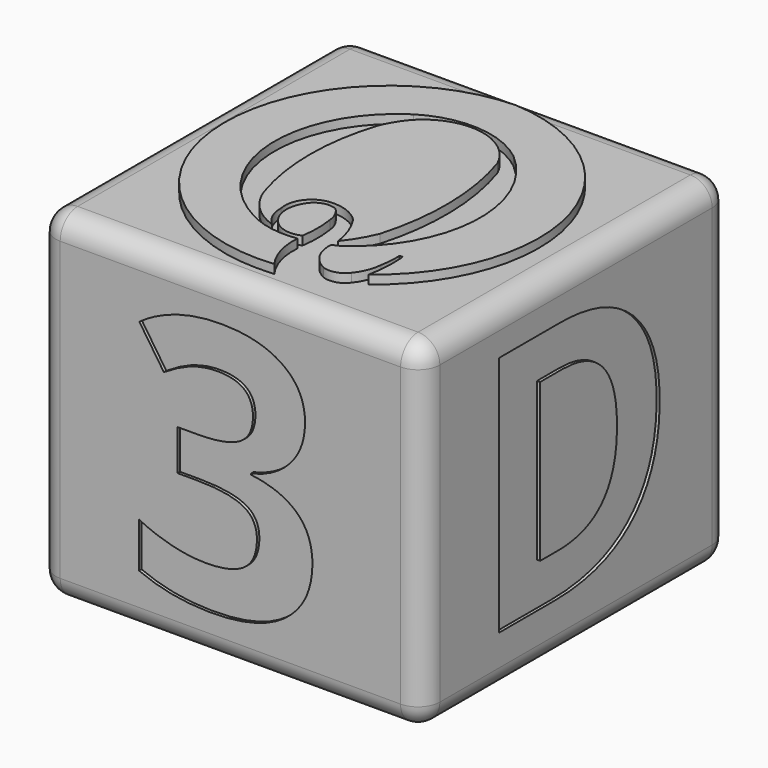
from build123d import *

# Parameters (mm, degrees)
F1_DEPTH      = 25
F4_DEPTH      = 55
F4_DEPTH_BACK = 23
F5_TEXT_SIZE  = 77.6406609496
F6_DEPTH      = 0.7
F7_TEXT_SIZE  = 80.3978016226
F8_DEPTH      = 0.7
F9_R          = 5


# Not quite as in the source:
# - Text() gives the source's letters only with a copy of the font that has no kerning and outlines rounded to 1/6400 em; it was checked with that copy


with BuildPart() as f1:
    # F0 (on Top) → F1 (new body)
    with BuildSketch(Plane.XY):
        with BuildLine():
            ThreePointArc((20.5675270408, -24.0095891058), (33.9110650067, 17.0205442488), (0, 43.6956547201))
            ThreePointArc((0, 43.6956547201), (-36.3351686492, 3.6568551313), (4.842115661, -31.3828539161))
            ThreePointArc((4.842115661, -31.3828539161), (2.4352442642, -26.4810804715), (1.9059170736, -21.0459884256))
            ThreePointArc((1.9059170736, -21.0459884256), (-4.1600004788, -20.9952833906), (-9.8727270961, -18.9550183713))
            ThreePointArc((-9.8727270961, -18.9550183713), (-24.8376639771, 4.6482965577), (-11.9922924787, 29.4688977301))
            ThreePointArc((-11.9922924787, 29.4688977301), (0.2712025373, 32.5646722625), (12.0852719992, 28.0474947466))
            ThreePointArc((12.0852719992, 28.0474947466), (22.4064776573, 5.6820438094), (12.0852719992, -16.6834071279))
            ThreePointArc((12.0852719992, -16.6834071279), (10.2163743213, -18.1512845309), (8.1104766577, -19.2524828017))
            ThreePointArc((8.1104766577, -19.2524828017), (9.1619138974, -23.770499049), (12.5694619492, -26.9179753959))
            ThreePointArc((12.5694619492, -26.9179753959), (15.3837710137, -27.0051807826), (17.7076142281, -25.4153087735))
            ThreePointArc((17.7076142281, -25.4153087735), (19.269837193, -22.7495971439), (19.9858490378, -19.7439547628))
            ThreePointArc((19.9858490378, -19.7439547628), (20.2921447856, -17.3055319325), (20.3251615167, -14.8481689394))
            Line((20.3251615167, -14.8481689394), (21.0256194399, -14.8481689394))
            Line((21.0256194399, -14.8481689394), (21.0522580892, -14.8481689394))
            ThreePointArc((21.0522580892, -14.8481689394), (21.0902538382, -15.2617533771), (21.1226022255, -15.6758177996))
            ThreePointArc((21.1226022255, -15.6758177996), (21.132303593, -19.8618351535), (20.5675270408, -24.0095891058))
        make_face()
        with BuildLine():
            ThreePointArc((21.0256194399, -14.8481689394), (21.0746144936, -15.2619343512), (21.1226022255, -15.6758177996))
            ThreePointArc((21.1226022255, -15.6758177996), (21.0902538382, -15.2617533771), (21.0522580892, -14.8481689394))
            Line((21.0522580892, -14.8481689394), (21.0256194399, -14.8481689394))
        make_face()
    extrude(amount=F1_DEPTH)



with BuildPart() as f1b:
    # F0 (on Top) → F1, piece 2 (new body)
    with BuildSketch(Plane.XY):
        with BuildLine():
            ThreePointArc((12.268330361, -10.3936661035), (14.5129050486, 6.9410317552), (11.5593973569, 24.1691093523))
            ThreePointArc((11.5593973569, 24.1691093523), (0.054070856, 31.9757142755), (-12.3297718844, 25.6546338853))
            ThreePointArc((-12.3297718844, 25.6546338853), (-13.3290953166, 23.9329823971), (-14.1917197034, 22.1389338089))
            ThreePointArc((-14.1917197034, 22.1389338089), (-16.7424053891, 5.8726338527), (-14.1917197034, -10.3936661035))
            ThreePointArc((-14.1917197034, -10.3936661035), (-10.7371054629, -16.0907978602), (-5.083876662, -19.6167975664))
            ThreePointArc((-5.083876662, -19.6167975664), (-7.0866938375, -16.9582762129), (-7.747025229, -13.6959189549))
            ThreePointArc((-7.747025229, -13.6959189549), (-6.7687697312, -8.9761092435), (-2.6743013877, -6.4327027649))
            ThreePointArc((-2.6743013877, -6.4327027649), (1.5733205373, -6.8874333521), (5.1653617993, -9.1996425763))
            ThreePointArc((5.1653617993, -9.1996425763), (7.1251059685, -13.0735291849), (8.192373784, -17.2816800941))
            ThreePointArc((8.192373784, -17.2816800941), (10.4826039511, -13.9869422067), (12.268330361, -10.3936661035))
        make_face()
    extrude(amount=F1_DEPTH)


with BuildPart() as f1c:
    # F0 (on Top) → F1, piece 3 (new body)
    with BuildSketch(Plane.XY):
        with BuildLine():
            ThreePointArc((-4.3943715282, -18.6494458467), (-1.3895715664, -20.0797383967), (1.9059170736, -19.6167975664))
            ThreePointArc((1.9059170736, -19.6167975664), (2.2170849753, -15.6672932208), (1.9059170736, -11.7177888751))
            ThreePointArc((1.9059170736, -11.7177888751), (1.2976371918, -9.5873136493), (0, -7.7914665453))
            ThreePointArc((0, -7.7914665453), (-3.1194388672, -7.6353877754), (-5.5577261373, -9.5873136493))
            ThreePointArc((-5.5577261373, -9.5873136493), (-6.6520631202, -14.3335387088), (-4.3943715282, -18.6494458467))
        make_face()
    extrude(amount=F1_DEPTH)


with BuildPart() as f1_1:
    add(f1.part)

    add(f1b.part)  # F4 merges F1b

    add(f1c.part)  # F4 merges F1c
    # F3 (on Top) → F4 (join, two sides)
    with BuildSketch(Plane.XY) as f4_sk:
        with BuildLine():
            Line((-39, -37.9130399376), (39, -37.9130399376))
            ThreePointArc((39, -37.9130399376), (42.5355339059, -36.4485738435), (44, -32.9130399376))
            Line((44, -32.9130399376), (44, 45.0869600624))
            ThreePointArc((44, 45.0869600624), (42.5355339059, 48.6224939683), (39, 50.0869600624))
            Line((39, 50.0869600624), (-39, 50.0869600624))
            ThreePointArc((-39, 50.0869600624), (-42.5355339059, 48.6224939683), (-44, 45.0869600624))
            Line((-44, 45.0869600624), (-44, -32.9130399376))
            ThreePointArc((-44, -32.9130399376), (-42.5355339059, -36.4485738435), (-39, -37.9130399376))
        make_face()
    extrude(amount=-F4_DEPTH)
    extrude(f4_sk.sketch, amount=F4_DEPTH_BACK)

    # F5 (on face) → F6 (cut)
    with BuildSketch(Plane.YZ.offset(44)):
        with Locations((-22.9130399376, -42.9012758837)):
            Text('D', F5_TEXT_SIZE, font='Open Sans', font_style=FontStyle.BOLD, text_align=(TextAlign.LEFT, TextAlign.BOTTOM))
    extrude(amount=-F6_DEPTH, mode=Mode.SUBTRACT)

    # F7 (on face) → F8 (cut)
    with BuildSketch(Plane.XZ.offset(37.9130399376)):
        with Locations((-24, -44.8864171683)):
            Text('3', F7_TEXT_SIZE, font='Open Sans', font_style=FontStyle.BOLD, text_align=(TextAlign.LEFT, TextAlign.BOTTOM))
    extrude(amount=-F8_DEPTH, mode=Mode.SUBTRACT)

    # F9
    f9_edges = [f1_1.edges().sort_by_distance(p)[0] for p in [
        (0, -37.91304, 23),
        (0, -37.91304, -55),
        (42.535534, -36.448574, -55),
        (44, 6.08696, -55),
        (42.535534, 48.622494, -55),
        (0, 50.08696, -55),
        (-42.535534, 48.622494, -55),
        (-44, 6.08696, -55),
        (-42.535534, -36.448574, -55),
    ]]
    fillet(f9_edges, radius=F9_R)


solid = f1_1.part
